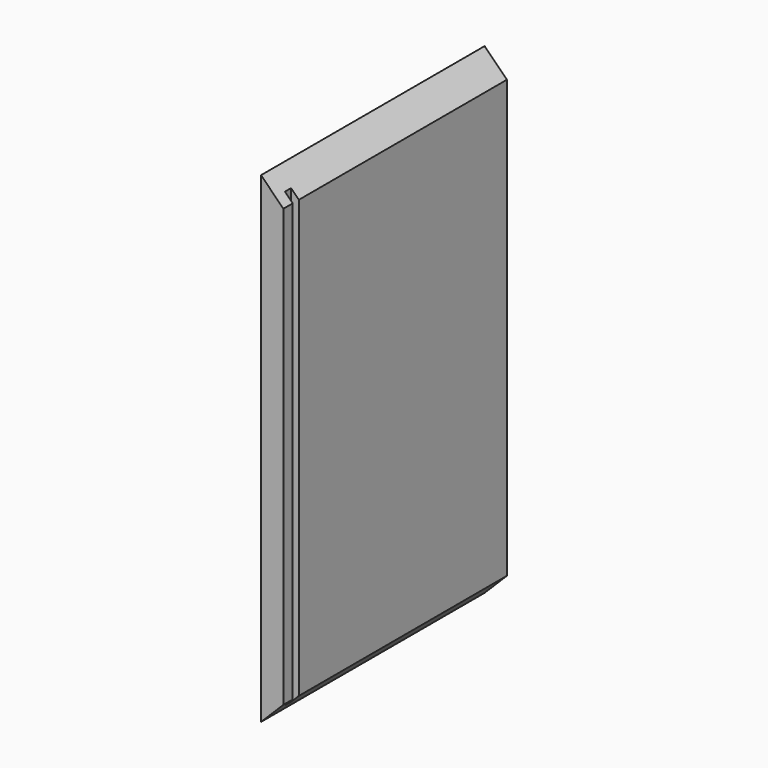
from build123d import *

# Parameters (mm, degrees)
F1_DEPTH = 196.85
F2_SIZE2 = 18.25624
F2_SIZE  = 18.25624
F3_SIZE  = 18.25624


# Not quite as in the source:
# - a fillet or chamfer is up to 0.001 mm smaller than in the source, because OpenCascade refuses the exact size


with BuildPart() as f1:
    # F0 (on Top) → F1 (new body, symmetric)
    with BuildSketch(Plane.XY):
        Polygon((9.128125, -98.425), (9.128125, 114.3), (-9.128125, 114.3), (-9.128125, -114.3), (9.128125, -114.3), (9.128125, -104.775), (2.778125, -104.775), (2.778125, -98.425), align=None)
    extrude(amount=F1_DEPTH, both=True)

    # F2 (size 18.25625 and 18.25625 in the source; OpenCascade refuses exactly that, so slightly less here)
    f2_edges = [f1.edges().sort_by_distance(p)[0] for p in [
        (9.128125, 7.9375, 196.85),
    ]]
    chamfer(f2_edges, length=F2_SIZE, length2=F2_SIZE2)

    # F3 (size 18.25625 in the source; OpenCascade refuses exactly that, so slightly less here)
    f3_edges = [f1.edges().sort_by_distance(p)[0] for p in [
        (9.128125, 7.9375, -196.85),
    ]]
    chamfer(f3_edges, length=F3_SIZE)


solid = f1.part
